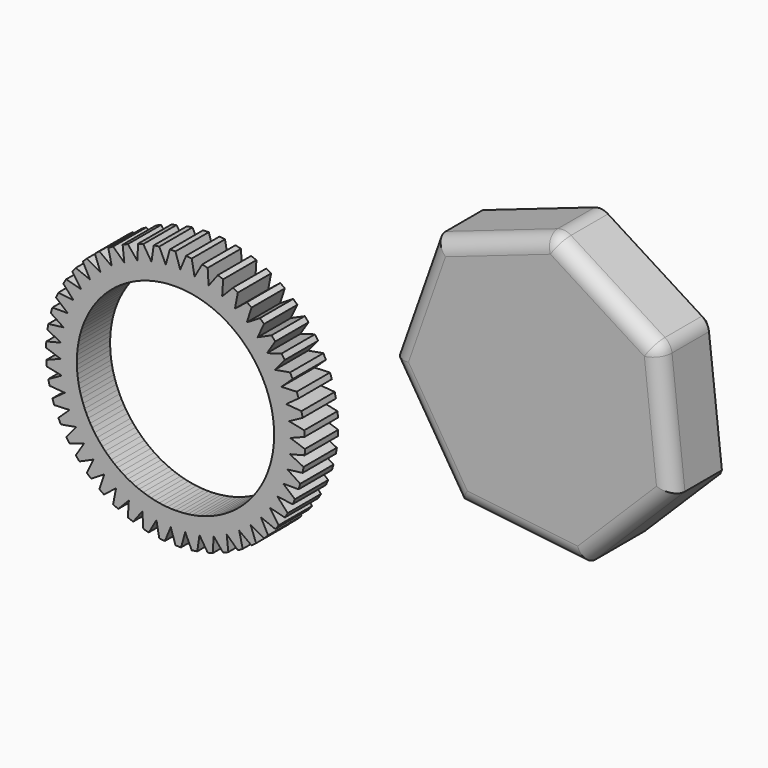
from build123d import *

# Parameters (mm, degrees)
F2_DEPTH     = 13.5
F3_COUNT     = 50
F5_DEPTH     = 25
F6_R         = 5
F7_T1_DEPTH  = 50.9610441595
F7_T3_DEPTH  = 65.8689172535
F7_T5_DEPTH  = 65.8689172535
F7_T7_DEPTH  = 65.8689172535
F7_T9_DEPTH  = 65.8689172535
F7_T11_DEPTH = 50.9610441595
F7_T13_DEPTH = 26.0196827351
F7_T18_DEPTH = 5
F7_T24_DEPTH = 5
F8_SIZE      = 4.99999


# Not quite as in the source:
# - a fillet or chamfer that OpenCascade refuses, or shapes differently, is made with other operations: its cross-section is extruded or revolved along the edge and cut away or added
# - a fillet or chamfer is up to 0.001 mm smaller than in the source, because OpenCascade refuses the exact size


with BuildPart() as f2:
    # F0 (on Front) → F2 (new body)
    with BuildSketch(Plane.XZ):
        with BuildLine():
            ThreePointArc((-1.3958203957, 31.9695430906), (-0.6980763211, 31.9923848666), (0, 32))
            ThreePointArc((0, 32), (0.7029915633, 31.9922772378), (1.4056438118, 31.9691126789))
            Line((1.4056438118, 31.9691126789), (1.6252756574, 36.9642865349))
            Line((1.6252756574, 36.9642865349), (0, 42))
            ThreePointArc((0, 42), (-0.9162251715, 41.9900051374), (-1.8320142693, 41.9600253064))
            Line((-1.8320142693, 41.9600253064), (-3.2360882882, 36.8582111963))
            Line((-3.2360882882, 36.8582111963), (-2.79877906, 31.8773718455))
            ThreePointArc((-2.79877906, 31.8773718455), (-2.0978060046, 31.9311636175), (-1.3958203957, 31.9695430906))
        make_face()
    extrude(amount=F2_DEPTH)

    # F3: F2 ×50 about axis
    f3_axis = Axis((0, -11.4520573989, 0), (0, -1, 0))


with BuildPart() as f2_1:
    add(f2.part)
    for i in range(1, F3_COUNT):
        add(f2.part.rotate(f3_axis, i * 360 / F3_COUNT))


with BuildPart() as f5:
    # F4 (on Front) → F5 (new body)
    with BuildSketch(Plane.XZ):
        Polygon((141.5398845793, 2.6642358221), (170.5213954329, 31.4798639797), (166.0621066118, 72.1047718649), (131.5199535513, 93.9475752431), (92.9058820374, 80.5601976585), (79.2970755036, 42.023607485), (100.9412428389, 7.3566431265), align=None)
    extrude(amount=F5_DEPTH)

    # F6
    f6_edges = [f5.edges().sort_by_distance(p)[0] for p in [
        (148.79103, -25, 83.026174),
    ]]
    fillet(f6_edges, radius=F6_R)

    # F7: fillet of radius 5 on 6 edges, made by hand

    # F7_s2 → F7_t1 (cut)
    with BuildSketch(Plane(origin=(-0.0202930617, 0, 0.1848733722), x_dir=(0, 1, 0), z_dir=(-0.1091119883, 0, 0.9940294634))):
        with BuildLine():
            ThreePointArc((-20, -172.9381217421), (-23.5355339059, -171.4736556481), (-25, -167.9381217421))
            Line((-25, -167.9381217421), (-25, -172.9381217421))
            Line((-25, -172.9381217421), (-20, -172.9381217421))
        make_face()
    extrude(amount=F7_T1_DEPTH, mode=Mode.SUBTRACT)

    # F7_s4 → F7_t3 (cut)
    with BuildSketch(Plane(origin=(63.6440999314, 0, 63.2798175125), x_dir=(0, 1, 0), z_dir=(0.709133317, 0, 0.7050744207))):
        with BuildLine():
            ThreePointArc((-25, -92.9068537416), (-23.5355339059, -96.4423876475), (-20, -97.9068537416))
            Line((-20, -97.9068537416), (-25, -97.9068537416))
            Line((-25, -97.9068537416), (-25, -92.9068537416))
        make_face()
    extrude(amount=F7_T3_DEPTH, mode=Mode.SUBTRACT)

    # F7_s6 → F7_t5 (cut)
    with BuildSketch(Plane(origin=(86.3541530083, 0, -9.9808476582), x_dir=(0, 1, 0), z_dir=(0.9933867709, 0, -0.1148160416))):
        with BuildLine():
            ThreePointArc((-25, 23.897665899), (-23.5355339059, 20.3621319931), (-20, 18.897665899))
            Line((-20, 18.897665899), (-25, 18.897665899))
            Line((-25, 18.897665899), (-25, 23.897665899))
        make_face()
    extrude(amount=F7_T5_DEPTH, mode=Mode.SUBTRACT)

    # F7_s8 → F7_t7 (cut)
    with BuildSketch(Plane(origin=(-3.2574187186, 0, 5.2173325437), x_dir=(0, 1, 0), z_dir=(0.5295997249, 0, -0.8482476828))):
        with BuildLine():
            ThreePointArc((-25, 94.5192515124), (-23.5355339059, 90.9837176064), (-20, 89.5192515124))
            Line((-20, 89.5192515124), (-25, 89.5192515124))
            Line((-25, 89.5192515124), (-25, 94.5192515124))
        make_face()
    extrude(amount=F7_T7_DEPTH, mode=Mode.SUBTRACT)

    # F7_s10 → F7_t9 (cut)
    with BuildSketch(Plane(origin=(39.7583388114, 0, 112.585244338), x_dir=(0, 1, 0), z_dir=(-0.3329867158, 0, -0.9429315177))):
        with BuildLine():
            ThreePointArc((-25, 65.7784087138), (-23.5355339059, 62.2428748078), (-20, 60.7784087138))
            Line((-20, 60.7784087138), (-25, 60.7784087138))
            Line((-25, 60.7784087138), (-25, 65.7784087138))
        make_face()
    extrude(amount=F7_T9_DEPTH, mode=Mode.SUBTRACT)

    # F7_s12 → F7_t11 (cut)
    with BuildSketch(Plane(origin=(144.2090600602, 0, 49.9968291989), x_dir=(0, 1, 0), z_dir=(-0.9448273678, 0, -0.3275686875))):
        with BuildLine():
            ThreePointArc((-25, -40.6824216631), (-23.5355339059, -44.217955569), (-20, -45.6824216631))
            Line((-20, -45.6824216631), (-25, -45.6824216631))
            Line((-25, -45.6824216631), (-25, -40.6824216631))
        make_face()
    extrude(amount=F7_T11_DEPTH, mode=Mode.SUBTRACT)

    # F7_s14 → F7_t13 (cut)
    with BuildSketch(Plane.XZ.offset(-6.0196827351)):
        with BuildLine():
            ThreePointArc((133.5550728193, 92.6606632795), (131.4568527994, 93.4016284294), (129.2449291538, 93.158831414))
            Line((129.2449291538, 93.158831414), (131.5199535513, 93.9475752431))
            Line((131.5199535513, 93.9475752431), (133.5550728193, 92.6606632795))
        make_face()
        with BuildLine():
            ThreePointArc((166.3248344326, 69.7112750655), (165.5959255298, 71.8137137486), (164.0269873438, 73.3916838285))
            Line((164.0269873438, 73.3916838285), (166.0621066118, 72.1047718649))
            Line((166.0621066118, 72.1047718649), (166.3248344326, 69.7112750655))
        make_face()
    extrude(amount=F7_T13_DEPTH, mode=Mode.SUBTRACT)


with BuildPart() as f7_tool16:
    # F7_s17 → F7_t18 (new body)
    with BuildSketch(Plane.XZ.offset(20)):
        Polygon((130.8827725913, 88.434694575), (129.2449291538, 93.158831414), (131.5199535513, 93.9475752431), (133.5550728193, 92.6606632795), align=None)
    extrude(amount=F7_T18_DEPTH)

    # F7_s19 → F7_t20 (revolve, cut)
    with BuildSketch(Plane(origin=(130.8827725913, -20, 88.434694575), x_dir=(-0.1148160416, 0, -0.9933867709), z_dir=(-0.9933867709, 0, 0.1148160416))):
        with BuildLine():
            ThreePointArc((0, -5), (5, 0), (0, 5))
            Line((0, 5), (0, -5))
        make_face()
    revolve(axis=Axis((130.8827725913, -20, 88.434694575), (0, -1, 0)), mode=Mode.SUBTRACT)


with BuildPart() as f5_1:
    add(f5.part)

    # F7_t15: cut F7_tool16
    add(f7_tool16.part, mode=Mode.SUBTRACT)


with BuildPart() as f7_tool22:
    # F7_s23 → F7_t24 (new body)
    with BuildSketch(Plane.XZ.offset(20)):
        Polygon((161.3546871159, 69.165715124), (166.3248344326, 69.7112750655), (166.0621066118, 72.1047718649), (164.0269873438, 73.3916838285), align=None)
    extrude(amount=F7_T24_DEPTH)

    # F7_s25 → F7_t26 (revolve, cut)
    with BuildSketch(Plane(origin=(161.3546871159, -20, 69.165715124), x_dir=(-0.8482476828, 0, -0.5295997249), z_dir=(-0.5295997249, 0, 0.8482476828))):
        with BuildLine():
            ThreePointArc((0, -5), (5, 0), (0, 5))
            Line((0, 5), (0, -5))
        make_face()
    revolve(axis=Axis((161.3546871159, -20, 69.165715124), (0, -1, 0)), mode=Mode.SUBTRACT)


with BuildPart() as f5_2:
    add(f5_1.part)

    # F7_t21: cut F7_tool22
    add(f7_tool22.part, mode=Mode.SUBTRACT)

    # F8 (size 5 in the source; OpenCascade refuses exactly that, so slightly less here)
    f8_edges = [f5_2.edges().sort_by_distance(p)[0] for p in [
        (111.075406, 0, 86.859515),
        (148.79103, 0, 83.026174),
        (131.456853, 0, 93.401628),
        (165.595926, 0, 71.813714),
        (168.423115, 0, 50.59557),
    ]]
    chamfer(f8_edges, length=F8_SIZE)


solid = Compound([f2_1.part, f5_2.part])
